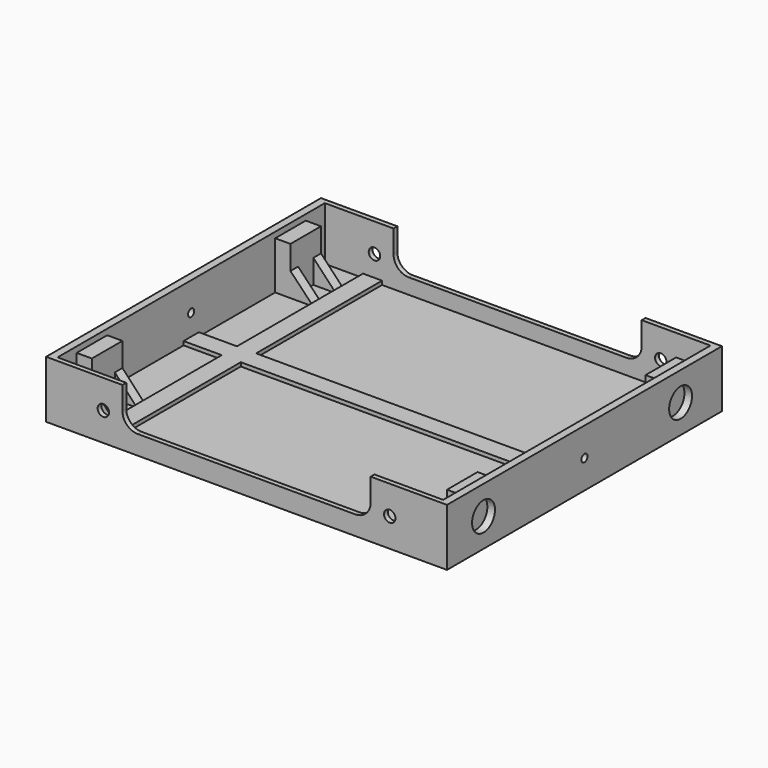
from build123d import *

# Parameters (mm, degrees)
F0_W      = 210
F0_H      = 180
F1_DEPTH  = 30
F2_W      = 202
F2_H      = 175
F3_DEPTH  = 28
F4_R      = 3
F5_DEPTH  = 4
F6_W      = 10
F6_H      = 82.5
F6_W_2    = 20
F6_H_2    = 10
F6_W_3    = 142
F7_DEPTH  = 2
F8_R      = 2
F9_DEPTH  = 5
F10_R     = 2
F10_R_2   = 7.5
F11_DEPTH = 5
F12_R     = 7.5
F13_DEPTH = 5
F14_W     = 8
F14_H     = 20
F15_DEPTH = 25
F17_DEPTH = 5
F19_DEPTH = 5
F21_DEPTH = 5
F23_DEPTH = 5
F25_DEPTH = 5
F27_DEPTH = 5
F30_DEPTH = 5
F32_DEPTH = 5
F33_R     = 3
F34_DEPTH = 4


# Not quite as in the source:
# - a feature names something its author has since deleted; it is built from what else it names


with BuildPart() as f1:
    # F0 (on Top) → F1 (new body)
    with BuildSketch(Plane.XY):
        Rectangle(F0_W, F0_H)
    extrude(amount=F1_DEPTH)

    # F2 (on face) → F3 (cut)
    with BuildSketch(Plane.XY.offset(30)):
        Rectangle(F2_W, F2_H)
    extrude(amount=-F3_DEPTH, mode=Mode.SUBTRACT)

    # F4 (on face) → F5 (cut)
    with BuildSketch(Plane.XZ.offset(90)):
        with BuildLine():
            Line((-57, 10), (-15, 10))
            Line((-15, 10), (15, 10))
            Line((15, 10), (57, 10))
            ThreePointArc((57, 10), (62.6568542495, 12.3431457505), (65, 18))
            Line((65, 18), (65, 30))
            Line((65, 30), (-65, 30))
            Line((-65, 30), (-65, 18))
            ThreePointArc((-65, 18), (-62.6568542495, 12.3431457505), (-57, 10))
        make_face()
        with Locations((-75, 15)):
            Circle(F4_R)
        with Locations((75, 15)):
            Circle(F4_R)
    extrude(amount=-F5_DEPTH, mode=Mode.SUBTRACT)

    # F8 (on face) → F9 (cut)
    with BuildSketch(Plane.YZ.offset(105)):
        with Locations((0, 15)):
            Circle(F8_R)
    extrude(amount=-F9_DEPTH, mode=Mode.SUBTRACT)

    # F10 (on face) → F11 (cut)
    with BuildSketch(Plane(origin=(-105, 0, 0), x_dir=(0, -1, 0), z_dir=(-1, 0, 0))):
        with Locations((0, 15)):
            Circle(F10_R)
        with Locations((-65, 15)):
            Circle(F10_R_2)
        with Locations((65, 15)):
            Circle(F10_R_2)
    extrude(amount=-F11_DEPTH, mode=Mode.SUBTRACT)

    # F12 (on face) → F13 (cut)
    with BuildSketch(Plane.YZ.offset(105)):
        with Locations((-66.0775899887, 15)):
            Circle(F12_R)
        with Locations((62.939658761, 15)):
            Circle(F12_R)
    extrude(amount=-F13_DEPTH, mode=Mode.SUBTRACT)

    # F14 (on face) → F15 (join)
    with BuildSketch(Plane.XY.offset(2)):
        with Locations((-97, 65)):
            Rectangle(F14_W, F14_H)
        with Locations((-97, -65)):
            Rectangle(F14_W, F14_H)
        with Locations((97, 65)):
            Rectangle(F14_W, F14_H)
        with Locations((97, -65)):
            Rectangle(F14_W, F14_H)
    extrude(amount=F15_DEPTH)

    # F16 (on face) → F17 (join)
    with BuildSketch(Plane(origin=(0, -55, 0), x_dir=(-1, 0, 0), z_dir=(0, 1, 0))):
        Polygon((-93, 2), (-81.6266089678, 1.707098214), (-93, 14.5), align=None)
    extrude(amount=-F17_DEPTH)

    # F18 (on face) → F19 (join)
    with BuildSketch(Plane.XZ.offset(-55)):
        Polygon((-93, 14.5), (-93, 2), (-81.0206457973, 2), align=None)
    extrude(amount=-F19_DEPTH)

    # F20 (on face) → F21 (join)
    with BuildSketch(Plane.XZ.offset(-55)):
        Polygon((81.1605315804, 2), (93, 2), (93, 14.5), align=None)
    extrude(amount=-F21_DEPTH)

    # F22 (on face) → F23 (join)
    with BuildSketch(Plane(origin=(0, -55, 0), x_dir=(-1, 0, 0), z_dir=(0, 1, 0))):
        Polygon((81.4045146108, 2), (93, 2), (93, 14.5), align=None)
    extrude(amount=-F23_DEPTH)

    # F24 (on face) → F25 (join)
    with BuildSketch(Plane(origin=(0, 75, 0), x_dir=(-1, 0, 0), z_dir=(0, 1, 0))):
        Polygon((81.214748323, 2), (93, 2), (93, 14.5), align=None)
    extrude(amount=-F25_DEPTH)

    # F26 (on face) → F27 (join)
    with BuildSketch(Plane.XZ.offset(75)):
        Polygon((81.2978520989, 2), (93, 2), (93, 14.5), align=None)
    extrude(amount=-F27_DEPTH)


with BuildPart() as f7:
    # F6 (on face) → F7 (new body)
    with BuildSketch(Plane.XY.offset(2)):
        with Locations((-76, 46.25)):
            Rectangle(F6_W, F6_H)
        with Locations((76, 46.25)):
            Rectangle(F6_W, F6_H)
        with Locations((-91, 0)):
            Rectangle(F6_W_2, F6_H_2)
        with Locations((-76, 0)):
            Rectangle(F6_W, F6_H_2)
        with Locations((-76, -46.25)):
            Rectangle(F6_W, F6_H)
        Rectangle(F6_W_3, F6_H_2)
        with Locations((76, 0)):
            Rectangle(F6_W, F6_H_2)
        with Locations((76, -46.25)):
            Rectangle(F6_W, F6_H)
        with Locations((91, 0)):
            Rectangle(F6_W_2, F6_H_2)
    extrude(amount=F7_DEPTH)


with BuildPart() as f1_1:
    add(f1.part)

    # F28: union F7
    add(f7.part)

    # F29 (on face) → F30 (join)
    with BuildSketch(Plane.XZ.offset(75)):
        Polygon((-93, 14.5), (-93, 2), (-81.4201831818, 2), align=None)
    extrude(amount=-F30_DEPTH)

    # F31 (on face) → F32 (join)
    with BuildSketch(Plane(origin=(0, 75, 0), x_dir=(-1, 0, 0), z_dir=(0, 1, 0))):
        Polygon((-93, 14.5), (-93, 2), (-81.2787339091, 2), align=None)
    extrude(amount=-F32_DEPTH)

    # F33 (on face) → F34 (cut)
    with BuildSketch(Plane(origin=(0, 90, 0), x_dir=(-1, 0, 0), z_dir=(0, 1, 0))):
        with BuildLine():
            Line((-57, 10.0647527289), (-15, 10.0647527289))
            Line((-15, 10.0647527289), (15, 10.0647527289))
            Line((15, 10.0647527289), (57, 10.0647527289))
            ThreePointArc((57, 10.0647527289), (62.6568542495, 12.4078984794), (65, 18.0647527289))
            Line((65, 18.0647527289), (65, 30))
            Line((65, 30), (-65, 30))
            Line((-65, 30), (-65, 18.0647527289))
            ThreePointArc((-65, 18.0647527289), (-62.6568542495, 12.4078984794), (-57, 10.0647527289))
        make_face()
        with Locations((-74.9857133275, 14.9857269089)):
            Circle(F33_R)
        with Locations((75, 15)):
            Circle(F33_R)
    extrude(amount=-F34_DEPTH, mode=Mode.SUBTRACT)


solid = f1_1.part
